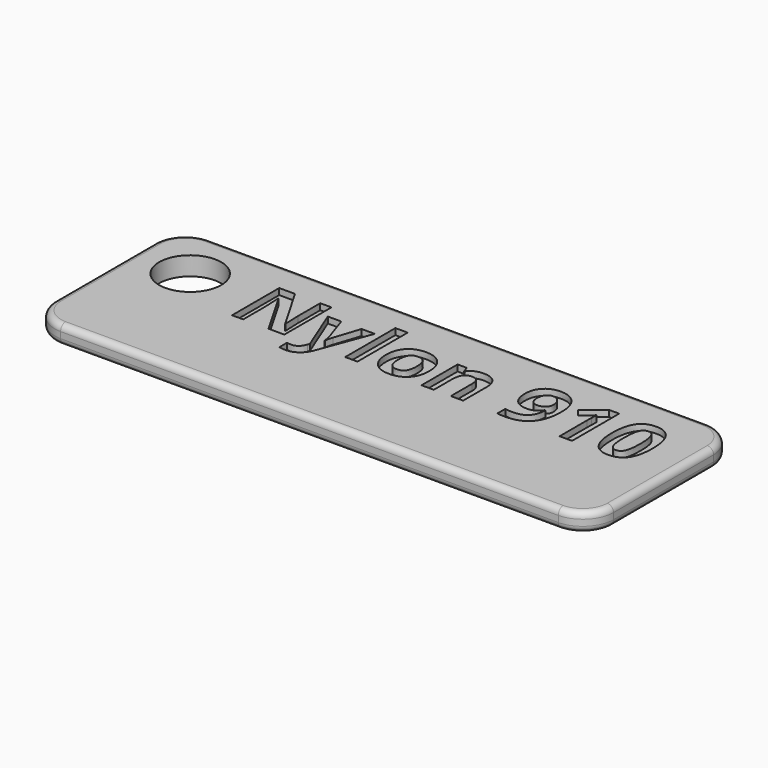
from build123d import *

# Parameters (mm, degrees)
F0_W         = 90
F0_H         = 30
F1_DEPTH     = 3
F2_R         = 1
F3_T1_DEPTH  = 3
F3_T4_ANGLE  = 90
F3_T6_ANGLE  = 90
F3_T8_ANGLE  = 90
F3_T10_ANGLE = 90
F3_T12_ANGLE = 90
F3_T14_ANGLE = 90
F3_T16_ANGLE = 90
F3_T18_ANGLE = 90
F4_R         = 5
F5_DEPTH     = 3
F6_TEXT_SIZE = 13.2934697089
F7_DEPTH     = 1


# Not quite as in the source:
# - a fillet or chamfer that OpenCascade refuses, or shapes differently, is made with other operations: its cross-section is extruded or revolved along the edge and cut away or added
# - Text() gives the source's letters only with a copy of the font that has no kerning and outlines rounded to 1/6400 em; it was checked with that copy


with BuildPart() as f1:
    # F0 (on Top) → F1 (new body)
    with BuildSketch(Plane.XY):
        Rectangle(F0_W, F0_H)
    extrude(amount=F1_DEPTH)

    # F2
    f2_edges = [f1.edges().sort_by_distance(p)[0] for p in [
        (0, 15, 3),
        (-45, 0, 3),
        (0, -15, 3),
        (45, 0, 3),
        (0, 15, 0),
        (-45, 0, 0),
        (0, -15, 0),
        (45, 0, 0),
    ]]
    fillet(f2_edges, radius=F2_R)

    # F3: fillet of radius 5 on 4 edges, made by hand

    # F3_s2 → F3_t1 (cut)
    with BuildSketch(Plane.XY):
        with BuildLine():
            ThreePointArc((45.0004, -9.9990343146), (43.5355339059, -13.5355339059), (39.9990343146, -15.0004))
            Line((39.9990343146, -15.0004), (39.9990343146, -15.5005365685))
            ThreePointArc((39.9990343146, -15.5005365685), (42.4995171573, -15.5001365685), (45, -15.5001365685))
            Line((45, -15.5001365685), (45.5001365685, -15))
            ThreePointArc((45.5001365685, -15), (45.5001365685, -12.4995171573), (45.5005365685, -9.9990343146))
            Line((45.5005365685, -9.9990343146), (45.0004, -9.9990343146))
        make_face()
        with BuildLine():
            ThreePointArc((39.9990343146, 15.0004), (43.5355339059, 13.5355339059), (45.0004, 9.9990343146))
            Line((45.0004, 9.9990343146), (45.5005365685, 9.9990343146))
            ThreePointArc((45.5005365685, 9.9990343146), (45.5001365685, 12.4995171573), (45.5001365685, 15))
            Line((45.5001365685, 15), (45, 15.5001365685))
            ThreePointArc((45, 15.5001365685), (42.4995171573, 15.5001365685), (39.9990343146, 15.5005365685))
            Line((39.9990343146, 15.5005365685), (39.9990343146, 15.0004))
        make_face()
        with BuildLine():
            ThreePointArc((-39.9990343146, 15.0004), (-43.5355339059, 13.5355339059), (-45.0004, 9.9990343146))
            Line((-45.0004, 9.9990343146), (-45.5005365685, 9.9990343146))
            ThreePointArc((-45.5005365685, 9.9990343146), (-45.5001365685, 12.4995171573), (-45.5001365685, 15))
            Line((-45.5001365685, 15), (-45, 15.5001365685))
            ThreePointArc((-45, 15.5001365685), (-42.4995171573, 15.5001365685), (-39.9990343146, 15.5005365685))
            Line((-39.9990343146, 15.5005365685), (-39.9990343146, 15.0004))
        make_face()
        with BuildLine():
            ThreePointArc((-45.0004, -9.9990343146), (-43.5355339059, -13.5355339059), (-39.9990343146, -15.0004))
            Line((-39.9990343146, -15.0004), (-39.9990343146, -15.5005365685))
            ThreePointArc((-39.9990343146, -15.5005365685), (-42.4995171573, -15.5001365685), (-45, -15.5001365685))
            Line((-45, -15.5001365685), (-45.5001365685, -15))
            ThreePointArc((-45.5001365685, -15), (-45.5001365685, -12.4995171573), (-45.5005365685, -9.9990343146))
            Line((-45.5005365685, -9.9990343146), (-45.0004, -9.9990343146))
        make_face()
    extrude(amount=F3_T1_DEPTH, mode=Mode.SUBTRACT)

    # F3_s3 → F3_t4 (revolve, cut)
    with BuildSketch(Plane.YZ.offset(-39.9990343146)):
        with BuildLine():
            ThreePointArc((-14.0004, 0), (-14.7075067812, 0.2928932188), (-15.0004, 1))
            Line((-15.0004, 1), (-15.0004, 0))
            Line((-15.0004, 0), (-14.0004, 0))
        make_face()
    revolve(axis=Axis((-39.9990343146, -9.9990343146, 0), (0, 0, -1)), revolution_arc=F3_T4_ANGLE, mode=Mode.SUBTRACT)

    # F3_s5 → F3_t6 (revolve, cut)
    with BuildSketch(Plane.XZ.offset(9.9990343146)):
        with BuildLine():
            ThreePointArc((-44.0004, 3), (-44.7075067812, 2.7071067812), (-45.0004, 2))
            Line((-45.0004, 2), (-45.0004, 3))
            Line((-45.0004, 3), (-44.0004, 3))
        make_face()
    revolve(axis=Axis((-39.9990343146, -9.9990343146, 3), (0, 0, 1)), revolution_arc=F3_T6_ANGLE, mode=Mode.SUBTRACT)

    # F3_s7 → F3_t8 (revolve, cut)
    with BuildSketch(Plane.XZ.offset(-9.9990343146)):
        with BuildLine():
            ThreePointArc((-44.0004, 0), (-44.7075067812, 0.2928932188), (-45.0004, 1))
            Line((-45.0004, 1), (-45.0004, 0))
            Line((-45.0004, 0), (-44.0004, 0))
        make_face()
    revolve(axis=Axis((-39.9990343146, 9.9990343146, 0), (0, 0, -1)), revolution_arc=F3_T8_ANGLE, mode=Mode.SUBTRACT)

    # F3_s9 → F3_t10 (revolve, cut)
    with BuildSketch(Plane.YZ.offset(-39.9990343146)):
        with BuildLine():
            ThreePointArc((14.0004, 3), (14.7075067812, 2.7071067812), (15.0004, 2))
            Line((15.0004, 2), (15.0004, 3))
            Line((15.0004, 3), (14.0004, 3))
        make_face()
    revolve(axis=Axis((-39.9990343146, 9.9990343146, 3), (0, 0, 1)), revolution_arc=F3_T10_ANGLE, mode=Mode.SUBTRACT)

    # F3_s11 → F3_t12 (revolve, cut)
    with BuildSketch(Plane.YZ.offset(39.9990343146)):
        with BuildLine():
            ThreePointArc((14.0004, 0), (14.7075067812, 0.2928932188), (15.0004, 1))
            Line((15.0004, 1), (15.0004, 0))
            Line((15.0004, 0), (14.0004, 0))
        make_face()
    revolve(axis=Axis((39.9990343146, 9.9990343146, 0), (0, 0, -1)), revolution_arc=F3_T12_ANGLE, mode=Mode.SUBTRACT)

    # F3_s13 → F3_t14 (revolve, cut)
    with BuildSketch(Plane.XZ.offset(-9.9990343146)):
        with BuildLine():
            ThreePointArc((44.0004, 3), (44.7075067812, 2.7071067812), (45.0004, 2))
            Line((45.0004, 2), (45.0004, 3))
            Line((45.0004, 3), (44.0004, 3))
        make_face()
    revolve(axis=Axis((39.9990343146, 9.9990343146, 3), (0, 0, 1)), revolution_arc=F3_T14_ANGLE, mode=Mode.SUBTRACT)

    # F3_s15 → F3_t16 (revolve, cut)
    with BuildSketch(Plane.XZ.offset(9.9990343146)):
        with BuildLine():
            ThreePointArc((44.0004, 0), (44.7075067812, 0.2928932188), (45.0004, 1))
            Line((45.0004, 1), (45.0004, 0))
            Line((45.0004, 0), (44.0004, 0))
        make_face()
    revolve(axis=Axis((39.9990343146, -9.9990343146, 0), (0, 0, -1)), revolution_arc=F3_T16_ANGLE, mode=Mode.SUBTRACT)

    # F3_s17 → F3_t18 (revolve, cut)
    with BuildSketch(Plane.YZ.offset(39.9990343146)):
        with BuildLine():
            ThreePointArc((-14.0004, 3), (-14.7075067812, 2.7071067812), (-15.0004, 2))
            Line((-15.0004, 2), (-15.0004, 3))
            Line((-15.0004, 3), (-14.0004, 3))
        make_face()
    revolve(axis=Axis((39.9990343146, -9.9990343146, 3), (0, 0, 1)), revolution_arc=F3_T18_ANGLE, mode=Mode.SUBTRACT)

    # F4 (on face) → F5 (cut)
    with BuildSketch(Plane.XY.offset(3)):
        with Locations((-36, 6)):
            Circle(F4_R)
    extrude(amount=-F5_DEPTH, mode=Mode.SUBTRACT)

    # F6 (on face) → F7 (cut)
    with BuildSketch(Plane.XY.offset(3)):
        with Locations((-26, 0.4287018096)):
            Text('Nylon 910', F6_TEXT_SIZE, font='Open Sans', font_style=FontStyle.BOLD, text_align=(TextAlign.LEFT, TextAlign.BOTTOM))
    extrude(amount=-F7_DEPTH, mode=Mode.SUBTRACT)


solid = f1.part
